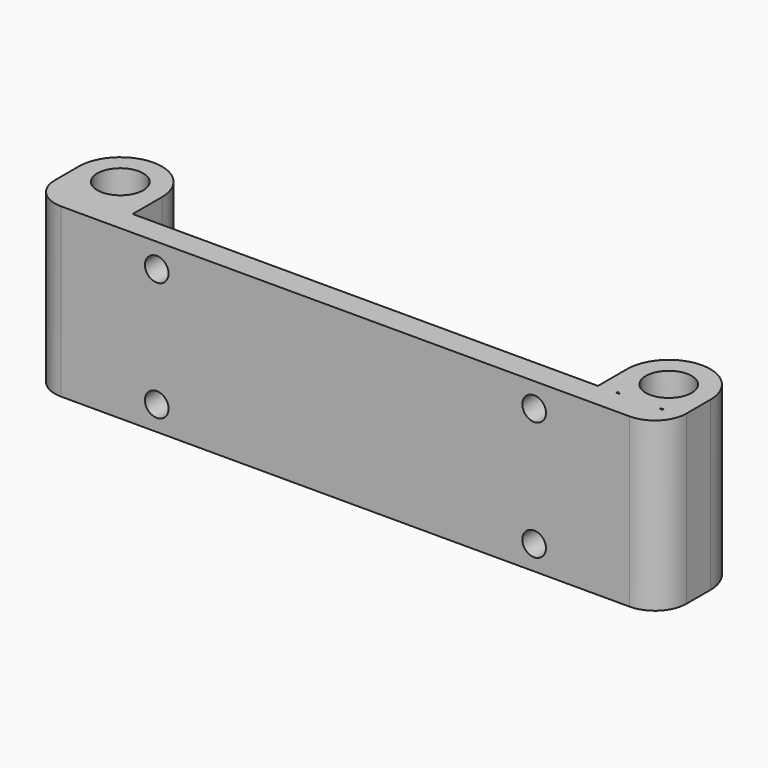
from build123d import *

# Parameters (mm, degrees)
F0_R     = 3.7
F1_DEPTH = 13.5
F2_R     = 5.08
F4_D     = 3.81


with BuildPart() as f1:
    # F0 (on Top) → F1 (new body, symmetric)
    with BuildSketch(Plane.XY):
        with BuildLine():
            Line((47.9, 2.3014477862), (47.9, 7.887150161))
            ThreePointArc((47.9, 7.887150161), (44.2, 4.187150161), (40.5, 7.887150161))
            Line((40.5, 7.887150161), (40.5, 2.3014477862))
            ThreePointArc((40.5, 2.3014477862), (40.7473700627, 2.1452499933), (41.0013230857, 2))
            Line((41.0013230857, 2), (47.3986769143, 2))
            ThreePointArc((47.3986769143, 2), (47.6526299373, 2.1452499933), (47.9, 2.3014477862))
        make_face()
        with BuildLine():
            ThreePointArc((40.5, 7.887150161), (44.2, 11.587150161), (47.9, 7.887150161))
            Line((47.9, 7.887150161), (47.9, 2.3014477862))
            ThreePointArc((47.9, 2.3014477862), (50.1025456639, 4.7169726099), (50.9000053, 7.887150161))
            ThreePointArc((50.9000053, 7.887150161), (44.2, 14.587155461), (37.4999947, 7.887150161))
            ThreePointArc((37.4999947, 7.887150161), (38.2974543361, 4.7169726099), (40.5, 2.3014477862))
            Line((40.5, 2.3014477862), (40.5, 7.887150161))
        make_face()
        with BuildLine():
            ThreePointArc((50.9000053, 7.887150161), (50.1025456639, 4.7169726099), (47.9, 2.3014477862))
            Line((47.9, 2.3014477862), (47.9, 2))
            Line((47.9, 2), (47.9, -2))
            Line((47.9, -2), (50.9000053, -2))
            Line((50.9000053, -2), (50.9000053, 7.887150161))
        make_face()
        with BuildLine():
            Line((40.5, 2), (40.5, 2.3014477862))
            ThreePointArc((40.5, 2.3014477862), (38.2974543361, 4.7169726099), (37.4999947, 7.887150161))
            Line((37.4999947, 7.887150161), (37.4999947, 2))
            Line((37.4999947, 2), (40.5, 2))
        make_face()
        with BuildLine():
            Line((47.9, -2), (47.9, 2))
            Line((47.9, 2), (47.3986769143, 2))
            ThreePointArc((47.3986769143, 2), (44.2, 1.187144861), (41.0013230857, 2))
            Line((41.0013230857, 2), (40.5, 2))
            Line((40.5, 2), (37.4999947, 2))
            Line((37.4999947, 2), (0, 2))
            Line((0, 2), (0, -2))
            Line((0, -2), (47.9, -2))
        make_face()
        with BuildLine():
            ThreePointArc((41.0013230857, 2), (44.2, 1.187144861), (47.3986769143, 2))
            Line((47.3986769143, 2), (41.0013230857, 2))
        make_face()
        with BuildLine():
            Line((-47.9, -2), (0, -2))
            Line((0, -2), (0, 2))
            Line((0, 2), (-37.4999947, 2))
            Line((-37.4999947, 2), (-41.0013230857, 2))
            ThreePointArc((-41.0013230857, 2), (-44.2, 1.187144861), (-47.3986769143, 2))
            ThreePointArc((-47.3986769143, 2), (-49.958525128, 4.4623203301), (-50.9000053, 7.887150161))
            Line((-50.9000053, 7.887150161), (-50.9000053, -2))
            Line((-50.9000053, -2), (-47.9, -2))
        make_face()
        with BuildLine():
            Line((-41.0013230857, 2), (-37.4999947, 2))
            Line((-37.4999947, 2), (-37.4999947, 7.887150161))
            ThreePointArc((-37.4999947, 7.887150161), (-38.441474872, 4.4623203301), (-41.0013230857, 2))
        make_face()
        with BuildLine():
            ThreePointArc((-47.3986769143, 2), (-44.2, 1.187144861), (-41.0013230857, 2))
            Line((-41.0013230857, 2), (-47.3986769143, 2))
        make_face()
        with BuildLine():
            Line((-47.3986769143, 2), (-41.0013230857, 2))
            ThreePointArc((-41.0013230857, 2), (-38.441474872, 4.4623203301), (-37.4999947, 7.887150161))
            ThreePointArc((-37.4999947, 7.887150161), (-44.2, 14.587155461), (-50.9000053, 7.887150161))
            ThreePointArc((-50.9000053, 7.887150161), (-49.958525128, 4.4623203301), (-47.3986769143, 2))
        make_face()
        with Locations((-44.2, 7.887150161)):
            Circle(F0_R, mode=Mode.SUBTRACT)
    extrude(amount=F1_DEPTH, both=True)

    # F2
    f2_edges = [f1.edges().sort_by_distance(p)[0] for p in [
        (50.900005, -2, 0),
        (-50.900005, -2, 0),
    ]]
    fillet(f2_edges, radius=F2_R)

    # F4 (through all)
    with Locations(Plane.XZ.offset(2)):
        with Locations((-30.41523, 9.59459), (-30.41523, -9.59459), (30.41523, -9.59459), (30.41523, 9.59459)):
            Hole(F4_D / 2)


solid = f1.part
